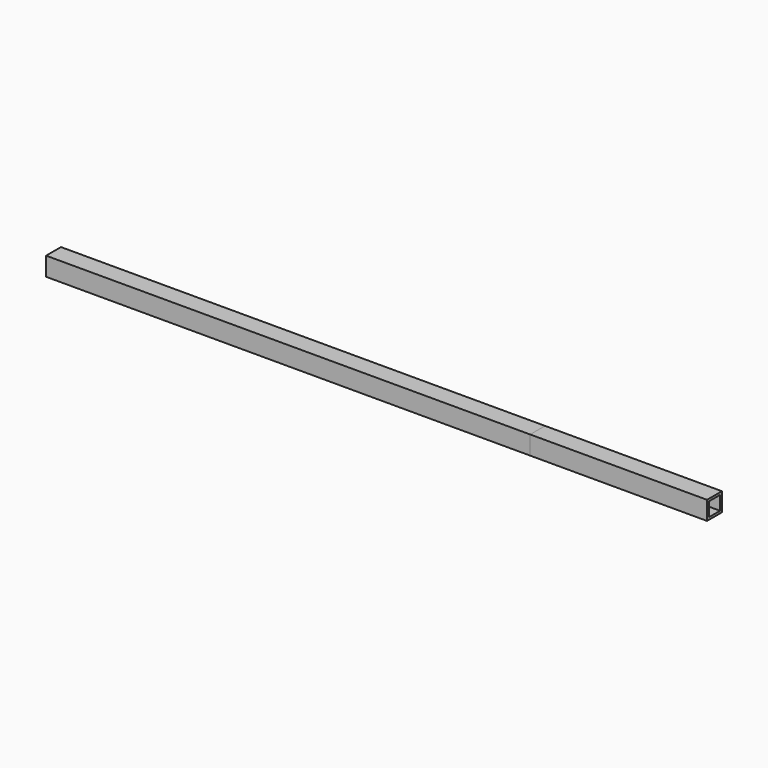
from build123d import *

# Parameters (mm, degrees)
F0_W     = 25.4
F0_H     = 25.4
F0_W_2   = 19.05
F0_H_2   = 19.05
F1_DEPTH = 901.7
F2_W     = 25.4
F2_H     = 25.4
F2_W_2   = 19.05
F2_H_2   = 19.05
F3_DEPTH = 353.3902
F5_DEPTH = 25.4
F6_W     = 25.4
F6_H     = 25.4
F6_W_2   = 19.05
F6_H_2   = 19.05
F7_DEPTH = 660.4


with BuildPart() as f1:
    # F0 (on Right) → F1 (new body)
    with BuildSketch(Plane.YZ):
        with Locations((12.7, 12.7)):
            Rectangle(F0_W, F0_H)
        with Locations((12.7, 12.7)):
            Rectangle(F0_W_2, F0_H_2, mode=Mode.SUBTRACT)
    extrude(amount=F1_DEPTH)


with BuildPart() as f3:
    # F2 (on Right) → F3 (new body)
    with BuildSketch(Plane.YZ):
        with Locations((12.7, 12.7)):
            Rectangle(F2_W, F2_H)
        with Locations((12.7, 12.7)):
            Rectangle(F2_W_2, F2_H_2, mode=Mode.SUBTRACT)
    extrude(amount=F3_DEPTH)

    # F4 (on face) → F5 (cut, through all)
    with BuildSketch(Plane.XZ):
        Polygon((340.7051866577, 25.4), (353.3902, 0), (353.3902, 25.4), align=None)
        Polygon((12.6850133423, 0), (0, 25.4), (0, 0), align=None)
    extrude(amount=-F5_DEPTH, mode=Mode.SUBTRACT)


with BuildPart() as f7:
    # F6 (on Right) → F7 (new body)
    with BuildSketch(Plane.YZ):
        with Locations((12.7, 12.7)):
            Rectangle(F6_W, F6_H)
        with Locations((12.7, 12.7)):
            Rectangle(F6_W_2, F6_H_2, mode=Mode.SUBTRACT)
    extrude(amount=F7_DEPTH)


solid = Compound([f1.part, f3.part, f7.part])
